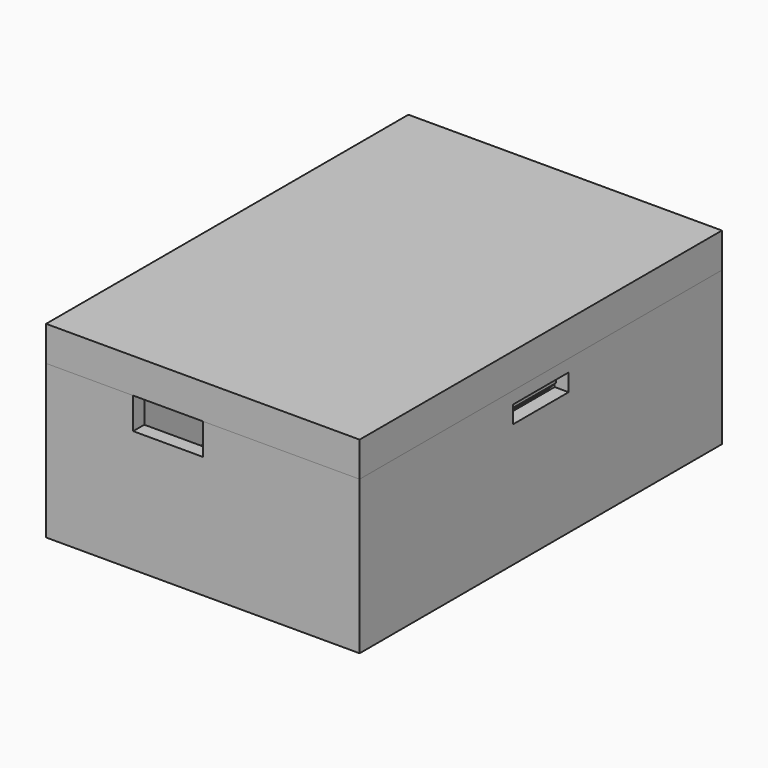
from build123d import *

# Parameters (mm, degrees)
F0_W      = 45
F0_H      = 65
F1_DEPTH  = 2
F2_W      = 45
F2_H      = 65
F2_W_2    = 41
F2_H_2    = 61
F3_DEPTH  = 20
F4_R      = 0.75
F5_DEPTH  = 5
F6_R      = 1.5
F7_DEPTH  = 2.5
F8_W      = 10
F8_H      = 4.5
F9_DEPTH  = 2
F10_W     = 10
F10_H     = 5
F11_DEPTH = 2
F12_W     = 1
F12_H     = 1.0020786701
F14_W     = 45
F14_H     = 65
F14_W_2   = 43
F14_H_2   = 63
F15_DEPTH = 1
F16_W     = 45
F16_H     = 65
F16_W_2   = 41
F16_H_2   = 61
F17_DEPTH = 4
F18_W     = 41
F18_H     = 1
F19_DEPTH = 61
F21_DEPTH = 4
F22_W     = 1
F22_H     = 2.5
F23_DEPTH = 5
F24_W     = 10
F24_H     = 2.5
F25_DEPTH = 2


with BuildPart() as f1:
    # F0 (on Top) → F1 (new body)
    with BuildSketch(Plane.XY):
        Rectangle(F0_W, F0_H)
    extrude(amount=F1_DEPTH)

    # F2 (on face) → F3 (join)
    with BuildSketch(Plane.XY.offset(2)):
        Rectangle(F2_W, F2_H)
        Rectangle(F2_W_2, F2_H_2, mode=Mode.SUBTRACT)
    extrude(amount=F3_DEPTH)

    # F4 (on face) → F5 (join)
    with BuildSketch(Plane.XY.offset(2)):
        with Locations((-18, 28)):
            Circle(F4_R)
        with Locations((-18, -28)):
            Circle(F4_R)
        with Locations((18, 28)):
            Circle(F4_R)
        with Locations((18, -28)):
            Circle(F4_R)
    extrude(amount=F5_DEPTH)

    # F6 (on face) → F7 (join)
    with BuildSketch(Plane.XY.offset(2)):
        with Locations((-18, 28)):
            Circle(F6_R)
        with Locations((-18, -28)):
            Circle(F6_R)
        with Locations((18, 28)):
            Circle(F6_R)
        with Locations((18, -28)):
            Circle(F6_R)
    extrude(amount=F7_DEPTH)

    # F8 (on face) → F9 (cut, through all)
    with BuildSketch(Plane.XZ.offset(32.5)):
        with Locations((-5, 19.75)):
            Rectangle(F8_W, F8_H)
    extrude(amount=-F9_DEPTH, mode=Mode.SUBTRACT)

    # F10 (on face) → F11 (cut, through all)
    with BuildSketch(Plane(origin=(0, 32.5, 0), x_dir=(-1, 0, 0), z_dir=(0, 1, 0))):
        with Locations((-14, 9.5)):
            Rectangle(F10_W, F10_H)
    extrude(amount=-F11_DEPTH, mode=Mode.SUBTRACT)

    # F13: sweep along a path in F13_path
    with BuildLine(Plane(origin=(-20.5, 30.5, 22), x_dir=(0, -1, 0), z_dir=(0, 0, -1))) as f13_path:
        Line((61, -20.5), (61, -41))
        Line((61, -41), (0, -41))
        Line((0, -41), (0, 0))
        Line((0, 0), (61, 0))
        Line((61, 0), (61, -10.5))
    # F12 (on face) → F13 (sweep)
    with BuildSketch(Plane(origin=(0, -30.5, 0), x_dir=(-1, 0, 0), z_dir=(0, 1, 0))):
        with Locations((21, 22.5010393351)):
            Rectangle(F12_W, F12_H)
    sweep(path=f13_path.line, transition=Transition.RIGHT)

    # F22 (on Front) → F23 (cut, symmetric)
    with BuildSketch(Plane.XZ):
        with Locations((-21, 19)):
            Rectangle(F22_W, F22_H)
    extrude(amount=F23_DEPTH, both=True, mode=Mode.SUBTRACT)

    # F24 (on face) → F25 (cut)
    with BuildSketch(Plane.YZ.offset(22.5)):
        with Locations((0, 19)):
            Rectangle(F24_W, F24_H)
    extrude(amount=-F25_DEPTH, mode=Mode.SUBTRACT)


with BuildPart() as f15:
    # F14 (on face) → F15 (new body)
    with BuildSketch(Plane.XY.offset(22)):
        Rectangle(F14_W, F14_H)
        Rectangle(F14_W_2, F14_H_2, mode=Mode.SUBTRACT)
    extrude(amount=F15_DEPTH)

    # F16 (on face) → F17 (join)
    with BuildSketch(Plane.XY.offset(23)):
        Rectangle(F16_W, F16_H)
        Rectangle(F16_W_2, F16_H_2, mode=Mode.SUBTRACT)
    extrude(amount=F17_DEPTH)

    # F18 (on face) → F19 (join, through all)
    with BuildSketch(Plane(origin=(0, -30.5, 0), x_dir=(-1, 0, 0), z_dir=(0, 1, 0))):
        with Locations((0, 26.5)):
            Rectangle(F18_W, F18_H)
    extrude(amount=F19_DEPTH)

    # F20 (on Front) → F21 (join, symmetric)
    with BuildSketch(Plane.XZ):
        Polygon((-18.75, 23.25), (-20.5, 25), (-20.5, 23), (-20.25, 23), (-20.25, 20), (-21.5, 20), (-21.5, 19), (-20.25, 17.75), (-18.75, 17.75), align=None)
        Polygon((20.25, 23), (20.5, 23), (20.5, 25), (18.75, 23.25), (18.75, 17.75), (20.25, 17.75), (21.5, 19), (21.5, 20), (20.25, 20), align=None)
    extrude(amount=F21_DEPTH, both=True)


solid = Compound([f1.part, f15.part])
